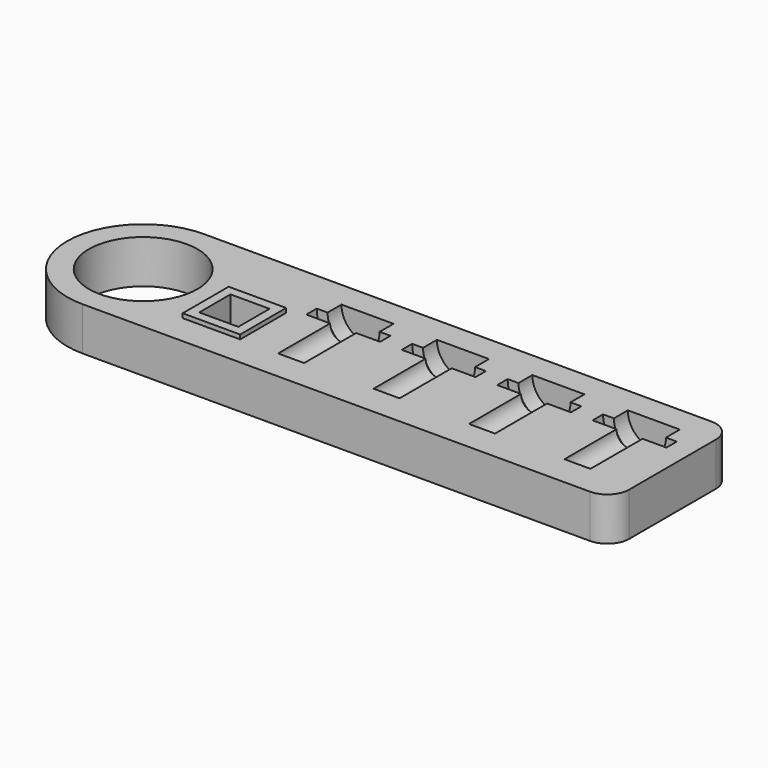
from build123d import *

# Parameters (mm, degrees)
F0_R         = 12.5
F1_DEPTH     = 10
F2_W         = 13.25
F2_H         = 13.25
F2_W_2       = 9
F2_H_2       = 9
F7_DEPTH     = 1
F8_DEPTH     = 5
F9_TEXT_SIZE = 5.5555555556
F10_DEPTH    = 1


# Not quite as in the source:
# - Text() gives the source's letters only with a copy of the font that has no kerning and outlines rounded to 1/6400 em; it was checked with that copy


with BuildPart() as f1:
    # F0 (on Top) → F1 (new body)
    with BuildSketch(Plane.XY):
        with BuildLine():
            ThreePointArc((0, 17.5), (5.1256313292, 5.1256313292), (17.5, 0))
            Line((17.5, 0), (134.5, 0))
            ThreePointArc((134.5, 0), (138.0355339059, 1.4644660941), (139.5, 5))
            Line((139.5, 5), (139.5, 30))
            ThreePointArc((139.5, 30), (138.0355339059, 33.5355339059), (134.5, 35))
            Line((134.5, 35), (17.5, 35))
            ThreePointArc((17.5, 35), (5.1256313292, 29.8743686708), (0, 17.5))
        make_face()
        with Locations((17.5, 17.5)):
            Circle(F0_R, mode=Mode.SUBTRACT)
    extrude(amount=F1_DEPTH)

    # F2 (on face) → F3 (revolve, cut)
    with BuildSketch(Plane.XY.offset(10)):
        Polygon((60, 22), (60, 7), (63, 7), (63, 22), (68.5, 22), (68.5, 25), (66, 25), (66, 29), (60, 29), (60, 25), align=None)
    revolve(axis=Axis((60, 14.5, 10), (0, 1, 0)), mode=Mode.SUBTRACT)

    # F2 (on face) → F4 (revolve, cut)
    with BuildSketch(Plane.XY.offset(10)):
        Polygon((82, 22), (82, 7), (85, 7), (85, 22), (90.5, 22), (90.5, 25), (88, 25), (88, 29), (82, 29), (82, 25), align=None)
    revolve(axis=Axis((82, 14.5, 10), (0, 1, 0)), mode=Mode.SUBTRACT)

    # F2 (on face) → F5 (revolve, cut)
    with BuildSketch(Plane.XY.offset(10)):
        Polygon((104, 22), (104, 7), (107, 7), (107, 22), (112.5, 22), (112.5, 25), (110, 25), (110, 29), (104, 29), (104, 25), align=None)
    revolve(axis=Axis((104, 14.5, 10), (0, 1, 0)), mode=Mode.SUBTRACT)

    # F2 (on face) → F6 (revolve, cut)
    with BuildSketch(Plane.XY.offset(10)):
        Polygon((126, 22), (126, 7), (129, 7), (129, 22), (134.5, 22), (134.5, 25), (132, 25), (132, 29), (126, 29), (126, 25), align=None)
    revolve(axis=Axis((126, 14.5, 10), (0, 1, 0)), mode=Mode.SUBTRACT)

    # F2 (on face) → F7 (join)
    with BuildSketch(Plane.XY.offset(10)):
        with Locations((41.625, 13.625)):
            Rectangle(F2_W, F2_H)
        with Locations((41.625, 13.625)):
            Rectangle(F2_W_2, F2_H_2, mode=Mode.SUBTRACT)
    extrude(amount=F7_DEPTH)

    # F2 (on face) → F8 (cut)
    with BuildSketch(Plane.XY.offset(10)):
        with Locations((41.625, 13.625)):
            Rectangle(F2_W_2, F2_H_2)
    extrude(amount=-F8_DEPTH, mode=Mode.SUBTRACT)

    # F9 (on face) → F10 (cut)
    with BuildSketch(Plane(origin=(0, 0, 0), x_dir=(1, 0, 0), z_dir=(0, 0, -1))):
        with Locations((30, -9)):
            Text('951, 952, 956', F9_TEXT_SIZE, font='Open Sans', text_align=(TextAlign.LEFT, TextAlign.BOTTOM))
    extrude(amount=-F10_DEPTH, mode=Mode.SUBTRACT)


solid = f1.part
